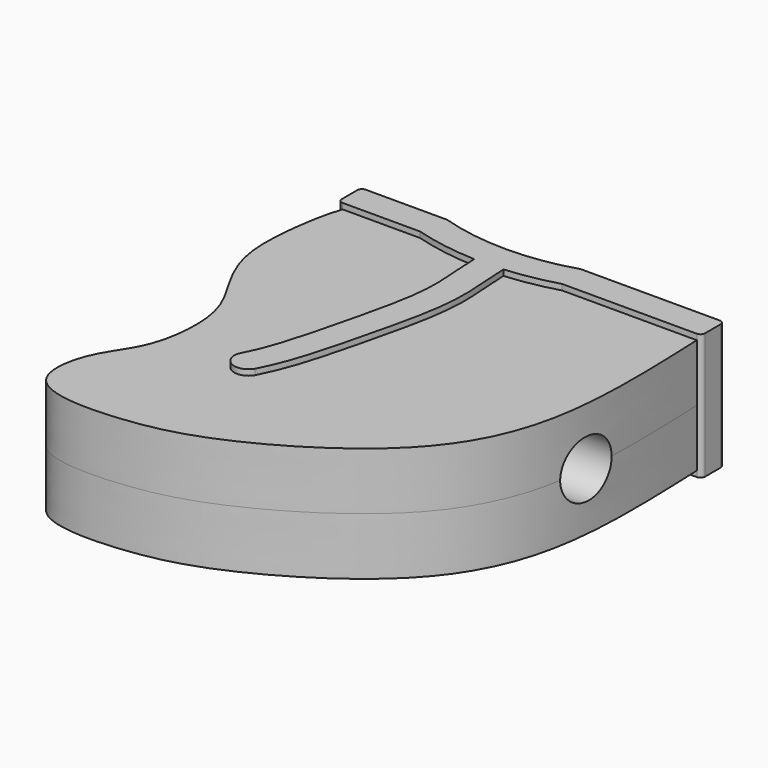
from build123d import *

# Parameters (mm, degrees)
F1_DEPTH = 6.985
F3_DEPTH = 6.35
F4_R     = 3.175
F5_DEPTH = 25.4


# Not quite as in the source:
# - the dataset's text gives a spline's control points without its knots; the knots are read off the source's solid


with BuildPart() as f1:
    # F0 (on Top) → F1 (new body, symmetric)
    with BuildSketch(Plane.XY):
        with BuildLine():
            Line((-8.5115687318, 0), (-17.5285687318, 0))
            ThreePointArc((-17.5285687318, 0), (-17.8877789767, -0.1487897552), (-18.0365687318, -0.508))
            Line((-18.0365687318, -0.508), (-18.0365687318, -2.667))
            ThreePointArc((-18.0365687318, -2.667), (-17.8877789767, -3.0262102448), (-17.5285687318, -3.175))
            Line((-17.5285687318, -3.175), (-8.9802561211, -3.175))
            ThreePointArc((-8.9802561211, -3.175), (-5.567721427, -3.9454225439), (-2.0857842173, -4.2846233733))
            ThreePointArc((-2.0857842173, -4.2846233733), (-0.4976584373, -4.2946352768), (1.0884838419, -4.2146577721))
            ThreePointArc((1.0884838419, -4.2146577721), (3.9459941464, -3.8405870368), (6.7499713132, -3.175))
            Line((6.7499713132, -3.175), (21.6482839239, -3.175))
            ThreePointArc((21.6482839239, -3.175), (22.0074941688, -3.0262102448), (22.1562839239, -2.667))
            Line((22.1562839239, -2.667), (22.1562839239, -0.508))
            ThreePointArc((22.1562839239, -0.508), (22.0074941688, -0.1487897552), (21.6482839239, 0))
            Line((21.6482839239, 0), (6.2812839239, 0))
            ThreePointArc((6.2812839239, 0), (-1.115142404, -1.1264395842), (-8.5115687318, 0))
        make_face()
        with BuildLine():
            ThreePointArc((1.0884838419, -4.2146577721), (-0.4976584373, -4.2946352768), (-2.0857842173, -4.2846233733))
            add(Edge.make_bspline(
                [(-2.0857842173, -4.2846233733), (-2.0186199799, -6.7917309713), (-1.3827408713, -10.7060362833), (-3.0514833549, -18.3702475343), (-5.3374183121, -27.5363695718), (-6.4696007178, -29.8358016288), (-6.9099617242, -30.7296345431)],
                knots=[0, 0, 0, 0, 0.2474193311, 0.5212563963, 0.8206566545, 1, 1, 1, 1], degree=3))
            ThreePointArc((-6.9099617242, -30.7296345431), (-6.1304191803, -32.7394350662), (-4.0618492346, -32.1328024756))
            add(Edge.make_bspline(
                [(1.0884838419, -4.2146577721), (1.1041136891, -4.7887191014), (1.1626428475, -5.8807272883), (1.2657335763, -7.2000093187), (1.3388942315, -8.2878331518), (1.379934699, -9.1286093049), (1.3942832103, -9.8573605503), (1.3885828158, -10.4588066051), (1.3694554964, -11.0762065107), (1.319036928, -11.8521658025), (1.1900459057, -13.0938268387), (0.9502096314, -14.6568714282), (0.5705234126, -16.567484773), (0.2002671656, -18.2057784722), (-0.1149929826, -19.5500794084), (-0.4435211016, -20.9313730655), (-0.8752970723, -22.6958190135), (-1.4129660983, -24.7785954156), (-1.867050274, -26.4097068901), (-2.230338473, -27.6119678291), (-2.5034145996, -28.4562408889), (-2.7788303173, -29.2346230816), (-3.1401362262, -30.1643913253), (-3.5830203882, -31.1620666475), (-3.9083126686, -31.8211580877), (-4.0618492346, -32.1328024756)],
                knots=[0.0005415805, 0.0005415805, 0.0005415805, 0.0005415805, 0.0625, 0.125, 0.15625, 0.1875, 0.21875, 0.234375, 0.25, 0.28125, 0.3125, 0.375, 0.4375, 0.5, 0.53125, 0.5625, 0.625, 0.6875, 0.75, 0.78125, 0.8125, 0.84375, 0.875, 0.9375, 1, 1, 1, 1], degree=3))
        make_face()
    extrude(amount=F1_DEPTH, both=True)

    # F2 (on Top) → F3 (join, symmetric)
    with BuildSketch(Plane.XY):
        with BuildLine():
            Line((-8.9802561211, -3.175), (-17.5285687318, -3.175))
            add(Edge.make_bspline(
                [(-17.5285687318, -3.175), (-18.2127580333, -4.9877029103), (-19.205941601, -11.3079780332), (-18.5687236072, -16.2930895041), (-16.5440340125, -20.3053098017), (-13.427143659, -25.0732944009), (-14.2177962554, -33.7662189884), (-17.9387187249, -37.5287065133), (-19.32437096, -46.023963295), (-7.2493815767, -46.1660242972), (2.3318830255, -43.5179077905), (16.3549608676, -34.7288777698), (22.463223389, -22.0953612128), (21.8986071096, -9.6631822871), (21.6482839239, -3.175)],
                knots=[0, 0, 0, 0, 0.0800290525, 0.1443448809, 0.2022093619, 0.2690099284, 0.3487252296, 0.4149445011, 0.4841972302, 0.5707600044, 0.663434281, 0.7748289004, 0.877945966, 1, 1, 1, 1], degree=3))
            Line((21.6482839239, -3.175), (6.7499713132, -3.175))
            ThreePointArc((6.7499713132, -3.175), (-1.115142404, -4.1752304513), (-8.9802561211, -3.175))
        make_face()
    extrude(amount=F3_DEPTH, both=True)

    # F4 (on Right) → F5 (cut, symmetric)
    with BuildSketch(Plane.YZ):
        with Locations((-18.3611052553, 0)):
            Circle(F4_R)
    extrude(amount=F5_DEPTH, both=True, mode=Mode.SUBTRACT)


solid = f1.part
